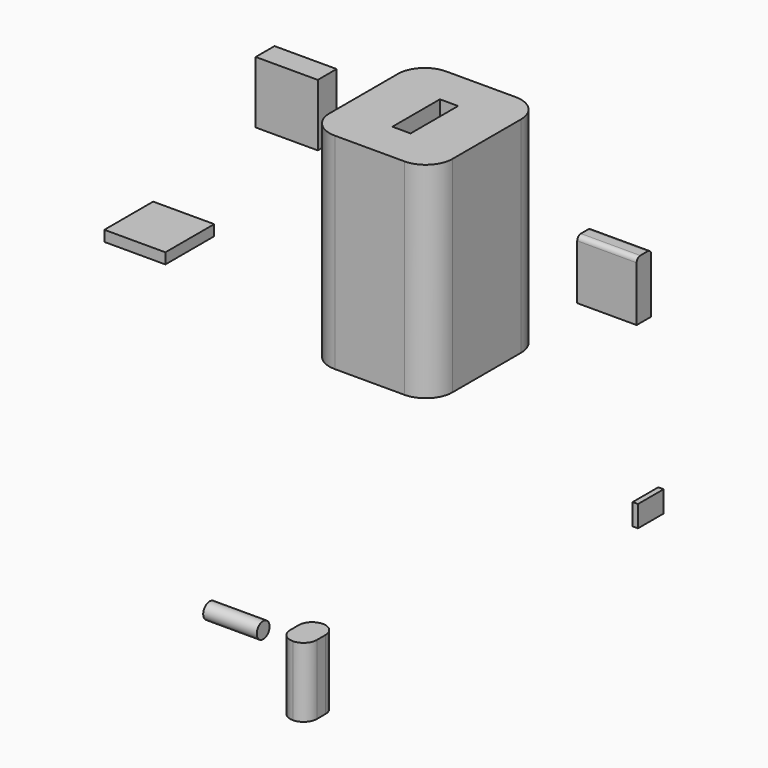
from build123d import *

# Parameters (mm, degrees)
F1_DEPTH      = 37.4
F2_DEPTH      = 1
F2_DEPTH_BACK = 1
F0_W          = 11.4
F0_H          = 11.4
F4_W          = 11.1
F4_H          = 3.4
F5_DEPTH      = 11.1
F6_W          = 11.6
F6_H          = 4.4
F7_DEPTH      = 11.6
F8_R          = 1.5
F9_DEPTH      = 10
F10_W         = 6
F10_H         = 4
F11_DEPTH     = 1
F12_W         = 7
F12_H         = 13
F13_DEPTH     = 5
F14_R         = 2.49999
F15_W         = 3.4
F15_H         = 11.1
F16_DEPTH     = 11.1
F17_R         = 0.85
F18_W         = 10
F18_H         = 1
F19_DEPTH     = 2


# Not quite as in the source:
# - a fillet or chamfer is up to 0.001 mm smaller than in the source, because OpenCascade refuses the exact size


with BuildPart() as f1:
    # F0 (on Top) → F1 (new body)
    with BuildSketch(Plane.XY):
        with BuildLine():
            ThreePointArc((11.5, 8), (10.0355339059, 11.5355339059), (6.5, 13))
            Line((6.5, 13), (-6.5, 13))
            ThreePointArc((-6.5, 13), (-10.0355339059, 11.5355339059), (-11.5, 8))
            Line((-11.5, 8), (-11.5, -8))
            ThreePointArc((-11.5, -8), (-10.0355339059, -11.5355339059), (-6.5, -13))
            Line((-6.5, -13), (6.5, -13))
            ThreePointArc((6.5, -13), (10.0355339059, -11.5355339059), (11.5, -8))
            Line((11.5, -8), (11.5, 8))
        make_face()
    extrude(amount=F1_DEPTH)

    # F0 (on Top) → F2 (join, two sides)
    with BuildSketch(Plane.XY) as f2_sk:
        with BuildLine():
            ThreePointArc((11.5, 8), (10.0355339059, 11.5355339059), (6.5, 13))
            Line((6.5, 13), (-6.5, 13))
            ThreePointArc((-6.5, 13), (-10.0355339059, 11.5355339059), (-11.5, 8))
            Line((-11.5, 8), (-11.5, -8))
            ThreePointArc((-11.5, -8), (-10.0355339059, -11.5355339059), (-6.5, -13))
            Line((-6.5, -13), (6.5, -13))
            ThreePointArc((6.5, -13), (10.0355339059, -11.5355339059), (11.5, -8))
            Line((11.5, -8), (11.5, 8))
        make_face()
    extrude(amount=F2_DEPTH)
    extrude(f2_sk.sketch, amount=-F2_DEPTH_BACK)

    # F15 (on face) → F16 (cut)
    with BuildSketch(Plane.XY.offset(37.4)):
        Rectangle(F15_W, F15_H)
    extrude(amount=-F16_DEPTH, mode=Mode.SUBTRACT)

    # F18 (on face) → F19 (cut)
    with BuildSketch(Plane(origin=(0, 0, -1), x_dir=(1, 0, 0), z_dir=(0, 0, -1))):
        with Locations((-1, -7)):
            Rectangle(F18_W, F18_H)
        with Locations((-1, 8)):
            Rectangle(F18_W, F18_H)
    extrude(amount=-F19_DEPTH, mode=Mode.SUBTRACT)


with BuildPart() as f2:
    # F0 (on Top) → F2, piece 2 (new body, two sides)
    with BuildSketch(Plane.XY) as f2_2_sk:
        with Locations((-52.1503757715, 3.0749998026)):
            Rectangle(F0_W, F0_H)
    extrude(amount=F2_DEPTH)
    extrude(f2_2_sk.sketch, amount=-F2_DEPTH_BACK)


with BuildPart() as f5:
    # F4 (on Top) → F5 (new body)
    with BuildSketch(Plane.XY):
        with Locations((14.8568219721, 25.5636378199)):
            Rectangle(F4_W, F4_H)
    extrude(amount=F5_DEPTH)

    # F17
    f17_edges = [f5.edges().sort_by_distance(p)[0] for p in [
        (14.856822, 27.263638, 11.1),
        (14.856822, 23.863638, 11.1),
    ]]
    fillet(f17_edges, radius=F17_R)


with BuildPart() as f7:
    # F6 (on Top) → F7 (new body)
    with BuildSketch(Plane.XY):
        with Locations((-56.1988651752, 40.1015764561)):
            Rectangle(F6_W, F6_H)
    extrude(amount=F7_DEPTH)


with BuildPart() as f9:
    # F8 (on Right) → F9 (new body)
    with BuildSketch(Plane.YZ):
        with Locations((-50.3522753716, -23.3863648027)):
            Circle(F8_R)
    extrude(amount=F9_DEPTH)


with BuildPart() as f11:
    # F10 (on Right) → F11 (new body)
    with BuildSketch(Plane.YZ):
        with Locations((51.4242419054, -47.7272756398)):
            Rectangle(F10_W, F10_H)
    extrude(amount=F11_DEPTH)


with BuildPart() as f13:
    # F12 (on Right) → F13 (new body)
    with BuildSketch(Plane.YZ):
        with Locations((-30.5454554036, -40.7653002545)):
            Rectangle(F12_W, F12_H)
    extrude(amount=F13_DEPTH)

    # F14 (radius 2.5 in the source; OpenCascade refuses exactly that, so slightly less here)
    f14_edges = [f13.edges().sort_by_distance(p)[0] for p in [
        (5, -34.045455, -40.7653),
        (5, -27.045455, -40.7653),
        (0, -27.045455, -40.7653),
        (0, -34.045455, -40.7653),
    ]]
    fillet(f14_edges, radius=F14_R)


solid = Compound([f1.part, f2.part, f5.part, f7.part, f9.part, f11.part, f13.part])
